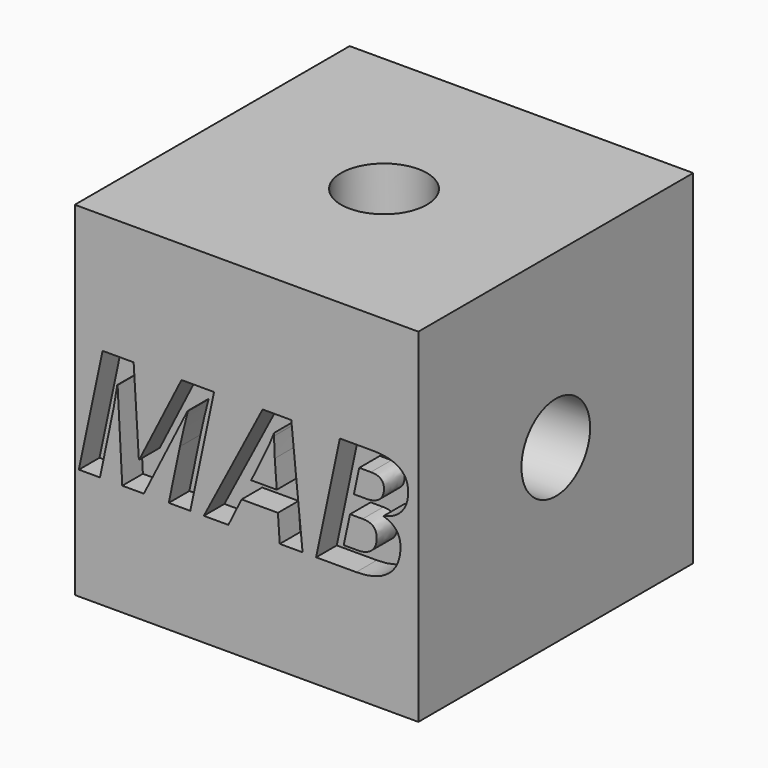
from build123d import *

# Parameters (mm, degrees)
F0_W         = 40
F0_H         = 40
F1_DEPTH     = 40
F2_TEXT_SIZE = 18.3197366538
F3_DEPTH     = 3
F4_R         = 5
F5_DEPTH     = 10
F6_R         = 5
F7_DEPTH     = 10
F8_R         = 5
F9_DEPTH     = 10
F10_R        = 5
F11_DEPTH    = 10


# Not quite as in the source:
# - Text() gives the source's letters only with a copy of the font that has no kerning and outlines rounded to 1/6400 em; it was checked with that copy


with BuildPart() as f1:
    # F0 (on Front) → F1 (new body)
    with BuildSketch(Plane.XZ):
        Rectangle(F0_W, F0_H)
    extrude(amount=F1_DEPTH)

    # F2 (on face) → F3 (cut)
    with BuildSketch(Plane.XZ.offset(40)):
        with Locations((-20, -7)):
            Text('MAB', F2_TEXT_SIZE, font='Open Sans', font_style=FontStyle.BOLDITALIC, text_align=(TextAlign.LEFT, TextAlign.BOTTOM))
    extrude(amount=-F3_DEPTH, mode=Mode.SUBTRACT)

    # F4 (on face) → F5 (cut)
    with BuildSketch(Plane.XY.offset(20)):
        with Locations((0, -20)):
            Circle(F4_R)
    extrude(amount=-F5_DEPTH, mode=Mode.SUBTRACT)

    # F6 (on face) → F7 (cut)
    with BuildSketch(Plane.YZ.offset(20)):
        with Locations((-20, 0)):
            Circle(F6_R)
    extrude(amount=-F7_DEPTH, mode=Mode.SUBTRACT)

    # F8 (on face) → F9 (cut)
    with BuildSketch(Plane(origin=(-20, 0, 0), x_dir=(0, -1, 0), z_dir=(-1, 0, 0))):
        with Locations((20, 0)):
            Circle(F8_R)
    extrude(amount=-F9_DEPTH, mode=Mode.SUBTRACT)

    # F10 (on face) → F11 (cut)
    with BuildSketch(Plane(origin=(0, 0, -20), x_dir=(1, 0, 0), z_dir=(0, 0, -1))):
        with Locations((0, 20)):
            Circle(F10_R)
    extrude(amount=-F11_DEPTH, mode=Mode.SUBTRACT)


solid = f1.part
